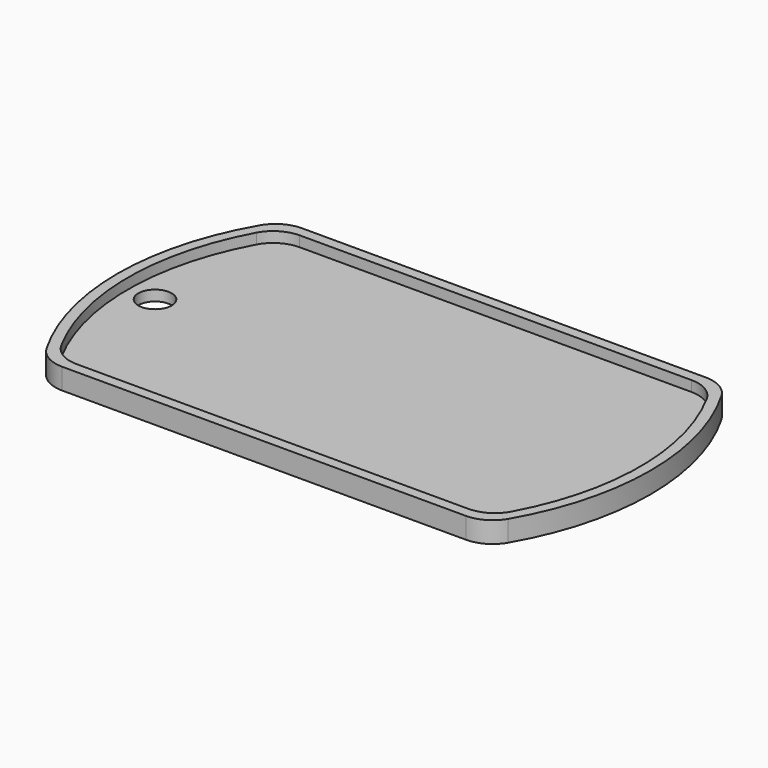
from build123d import *

# Parameters (mm, degrees)
F1_DEPTH = 1
F3_DEPTH = 1
F4_R     = 1.5875
F5_DEPTH = 1


# Not quite as in the source:
# - a feature of the source that left no trace in its solid (it failed there, or was rolled back) is left out


with BuildPart() as f1:
    # F0 (on Top) → F1 (new body)
    with BuildSketch(Plane.XY):
        with BuildLine():
            ThreePointArc((-19.2474145991, 14.2875), (-20.8349145991, 13.862130657), (-21.9970452561, 12.7))
            ThreePointArc((-21.9970452561, 12.7), (-25.4, 0), (-21.9970452561, -12.7))
            ThreePointArc((-21.9970452561, -12.7), (-20.8349145991, -13.862130657), (-19.2474145991, -14.2875))
            Line((-19.2474145991, -14.2875), (19.2474145991, -14.2875))
            ThreePointArc((19.2474145991, -14.2875), (20.8349145991, -13.862130657), (21.9970452561, -12.7))
            ThreePointArc((21.9970452561, -12.7), (25.4, 0), (21.9970452561, 12.7))
            ThreePointArc((21.9970452561, 12.7), (20.8349145991, 13.862130657), (19.2474145991, 14.2875))
            Line((19.2474145991, 14.2875), (-19.2474145991, 14.2875))
        make_face()
    extrude(amount=F1_DEPTH)

    # F2 (on face) → F3 (join)
    with BuildSketch(Plane.XY.offset(1)):
        with BuildLine():
            Line((19.2474145991, 14.2875), (-19.2474145991, 14.2875))
            ThreePointArc((-19.2474145991, 14.2875), (-20.8349145991, 13.862130657), (-21.9970452561, 12.7))
            ThreePointArc((-21.9970452561, 12.7), (-25.4, 0), (-21.9970452561, -12.7))
            ThreePointArc((-21.9970452561, -12.7), (-20.8349145991, -13.862130657), (-19.2474145991, -14.2875))
            Line((-19.2474145991, -14.2875), (19.2474145991, -14.2875))
            ThreePointArc((19.2474145991, -14.2875), (20.8349145991, -13.862130657), (21.9970452561, -12.7))
            ThreePointArc((21.9970452561, -12.7), (25.4, 0), (21.9970452561, 12.7))
            ThreePointArc((21.9970452561, 12.7), (20.8349145991, 13.862130657), (19.2474145991, 14.2875))
        make_face()
        with BuildLine():
            ThreePointArc((-21.4526124879, 11.6252061249), (-20.2856017842, 12.8404540819), (-18.6611352482, 13.2875))
            Line((-18.6611352482, 13.2875), (18.6611352482, 13.2875))
            ThreePointArc((18.6611352482, 13.2875), (20.2856017842, 12.8404540819), (21.4526124879, 11.6252061249))
            ThreePointArc((21.4526124879, 11.6252061249), (24.4, 0), (21.4526124879, -11.6252061249))
            ThreePointArc((21.4526124879, -11.6252061249), (20.2856017842, -12.8404540819), (18.6611352482, -13.2875))
            Line((18.6611352482, -13.2875), (-18.6611352482, -13.2875))
            ThreePointArc((-18.6611352482, -13.2875), (-20.2856017842, -12.8404540819), (-21.4526124879, -11.6252061249))
            ThreePointArc((-21.4526124879, -11.6252061249), (-24.4, 0), (-21.4526124879, 11.6252061249))
        make_face(mode=Mode.SUBTRACT)
    extrude(amount=F3_DEPTH)

    # F4 (on face) → F5 (cut)
    with BuildSketch(Plane.XY.offset(1)):
        with Locations((-21.821282804, 0)):
            Circle(F4_R)
    extrude(amount=-F5_DEPTH, mode=Mode.SUBTRACT)


solid = f1.part
